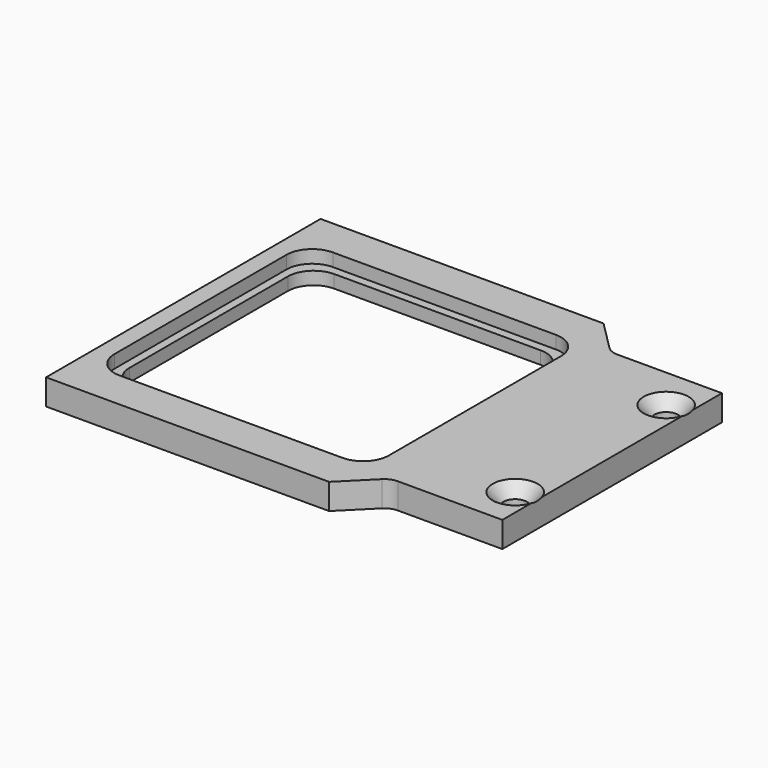
from build123d import *

# Parameters (mm, degrees)
F1_DEPTH       = 9.525
F3_DEPTH       = 4.7752
F4_DEPTH       = 9.526
F6_D           = 8.73125
F6_CSINK_D     = 16.6624
F6_CSINK_ANGLE = 82


# Not quite as in the source:
# - a length typed as a fraction of an inch, garbled in the dataset ("3 / 203.2 mm" for 3/8 in), is restored


with BuildPart() as f1:
    # F0 (on Top) → F1 (new body)
    with BuildSketch(Plane.XY):
        with BuildLine():
            Line((37.8966893194, 57.4490684102), (-66.8783106806, 57.4490684102))
            Line((-66.8783106806, 57.4490684102), (-66.8783106806, -69.5509315898))
            Line((-66.8783106806, -69.5509315898), (37.8966893194, -69.5509315898))
            Line((37.8966893194, -69.5509315898), (48.7368173799, -58.7108035293))
            ThreePointArc((48.7368173799, -58.7108035293), (50.796905645, -57.3342965584), (53.2269454405, -56.8509315898))
            Line((53.2269454405, -56.8509315898), (91.8716893194, -56.8509315898))
            Line((91.8716893194, -56.8509315898), (91.8716893194, 44.7490684102))
            Line((91.8716893194, 44.7490684102), (53.2269454405, 44.7490684102))
            ThreePointArc((53.2269454405, 44.7490684102), (50.796905645, 45.2324333787), (48.7368173799, 46.6089403496))
            Line((48.7368173799, 46.6089403496), (37.8966893194, 57.4490684102))
        make_face()
    extrude(amount=F1_DEPTH)

    # F2 (on face) → F3 (cut)
    with BuildSketch(Plane.XY.offset(9.525)):
        with BuildLine():
            Line((31.5466893194, 43.2885684102), (-51.0033106806, 43.2885684102))
            ThreePointArc((-51.0033106806, 43.2885684102), (-57.7385027714, 40.498760501), (-60.5283106806, 33.7635684102))
            Line((-60.5283106806, 33.7635684102), (-60.5283106806, -45.8654315898))
            ThreePointArc((-60.5283106806, -45.8654315898), (-57.7385027714, -52.6006236806), (-51.0033106806, -55.3904315898))
            Line((-51.0033106806, -55.3904315898), (31.5466893194, -55.3904315898))
            ThreePointArc((31.5466893194, -55.3904315898), (38.2818814102, -52.6006236806), (41.0716893194, -45.8654315898))
            Line((41.0716893194, -45.8654315898), (41.0716893194, 33.7635684102))
            ThreePointArc((41.0716893194, 33.7635684102), (38.2818814102, 40.498760501), (31.5466893194, 43.2885684102))
        make_face()
        with BuildLine():
            ThreePointArc((-57.4803106806, 30.5885684102), (-54.6905027714, 37.323760501), (-47.9553106806, 40.1135684102))
            Line((-47.9553106806, 40.1135684102), (28.4986893194, 40.1135684102))
            ThreePointArc((28.4986893194, 40.1135684102), (35.2338814102, 37.323760501), (38.0236893194, 30.5885684102))
            Line((38.0236893194, 30.5885684102), (38.0236893194, -42.6904315898))
            ThreePointArc((38.0236893194, -42.6904315898), (35.2338814102, -49.4256236806), (28.4986893194, -52.2154315898))
            Line((28.4986893194, -52.2154315898), (-47.9553106806, -52.2154315898))
            ThreePointArc((-47.9553106806, -52.2154315898), (-54.6905027714, -49.4256236806), (-57.4803106806, -42.6904315898))
            Line((-57.4803106806, -42.6904315898), (-57.4803106806, 30.5885684102))
        make_face(mode=Mode.SUBTRACT)
    extrude(amount=-F3_DEPTH, mode=Mode.SUBTRACT)

    # F4 (cut, through all): a face of the model
    f4_faces = [f1.faces().sort_by_distance(p)[0] for p in [
        (-9.7283106806, -6.0509315898, 9.525),
    ]]
    extrude(f4_faces, amount=-F4_DEPTH, mode=Mode.SUBTRACT)

    # F6 (through all)
    with Locations(Plane.XY.offset(9.525)):
        with Locations((83.9214893194, 28.8740684102), (83.9214893194, -40.9759315898)):
            CounterSinkHole(F6_D / 2, F6_CSINK_D / 2, counter_sink_angle=F6_CSINK_ANGLE)


solid = f1.part
